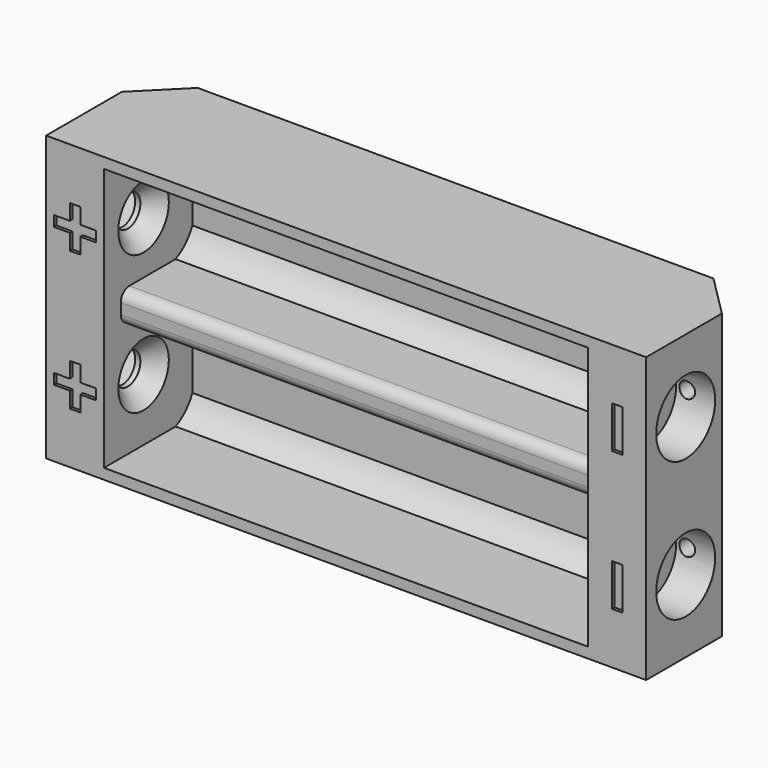
from build123d import *

# Parameters (mm, degrees)
F0_W          = 57
F0_H          = 27
F0_W_2        = 46
F0_H_2        = 25
F1_DEPTH      = 13
F2_DEPTH      = 2.5
F3_W          = 10
F3_H          = 3
F4_DEPTH      = 46
F5_R          = 1.5
F6_DEPTH      = 5.501
F6_DEPTH_BACK = 51.501
F7_SIZE       = 1.5
F8_R          = 1.5
F9_DEPTH      = 3.5
F10_R         = 3.5
F10_R_2       = 1.5
F11_DEPTH     = 3.7
F13_DEPTH     = 46
F14_R         = 1.2
F15_DEPTH     = 57.001
F16_R         = 0.75
F17_DEPTH     = 6
F18_T1_DEPTH  = 47.5734639037
F19_W         = 1
F19_H         = 4
F19_H_2       = 1.5
F19_W_2       = 1.5
F19_H_3       = 1
F20_DEPTH     = 0.3
F21_R         = 1


# Not quite as in the source:
# - a fillet or chamfer that OpenCascade refuses, or shapes differently, is made with other operations: its cross-section is extruded or revolved along the edge and cut away or added


with BuildPart() as f1:
    # F0 (on Front) → F1 (new body)
    with BuildSketch(Plane.XZ):
        Rectangle(F0_W, F0_H)
        Rectangle(F0_W_2, F0_H_2, mode=Mode.SUBTRACT)
    extrude(amount=F1_DEPTH)

    # F0 (on Front) → F2 (join)
    with BuildSketch(Plane.XZ):
        Rectangle(F0_W_2, F0_H_2)
    extrude(amount=F2_DEPTH)

    # F3 (on face) → F4 (join, through all)
    with BuildSketch(Plane.YZ.offset(-23)):
        with Locations((-6, 0)):
            Rectangle(F3_W, F3_H)
    extrude(amount=F4_DEPTH)

    # F5 (on face) → F6 (cut, two sides)
    with BuildSketch(Plane.YZ.offset(-23)) as f6_sk:
        with Locations((-8.3, 6.6)):
            Circle(F5_R)
        with Locations((-8.3, -6.6)):
            Circle(F5_R)
    extrude(amount=-F6_DEPTH, mode=Mode.SUBTRACT)
    extrude(f6_sk.sketch, amount=F6_DEPTH_BACK, mode=Mode.SUBTRACT)

    # F7
    f7_edges = [f1.edges().sort_by_distance(p)[0] for p in [
        (-23, -9.8, 6.6),
        (-23, -9.8, -6.6),
        (23, -9.8, 6.6),
        (23, -9.8, -6.6),
    ]]
    chamfer(f7_edges, length=F7_SIZE)

    # F8 (on face) → F9 (cut)
    with BuildSketch(Plane(origin=(-28.5, 0, 0), x_dir=(0, -1, 0), z_dir=(-1, 0, 0))):
        Polygon((6.5679491924, -3.6), (4.8358983849, -6.6), (6.5679491924, -9.6), (10.0320508076, -9.6), (11.7641016151, -6.6), (10.0320508076, -3.6), align=None)
        with Locations((8.3, -6.6)):
            Circle(F8_R, mode=Mode.SUBTRACT)
        Polygon((10.0320508076, 9.6), (6.5679491924, 9.6), (4.8358983849, 6.6), (6.5679491924, 3.6), (10.0320508076, 3.6), (11.7641016151, 6.6), align=None)
        with Locations((8.3, 6.6)):
            Circle(F8_R, mode=Mode.SUBTRACT)
        with Locations((8.3, 6.6)):
            Circle(F8_R)
    extrude(amount=-F9_DEPTH, mode=Mode.SUBTRACT)

    # F10 (on face) → F11 (cut)
    with BuildSketch(Plane.YZ.offset(28.5)):
        with Locations((-8.3, 6.6)):
            Circle(F10_R)
        with Locations((-8.3, 6.6)):
            Circle(F10_R_2, mode=Mode.SUBTRACT)
        with Locations((-8.3, -6.6)):
            Circle(F10_R)
        with Locations((-8.3, -6.6)):
            Circle(F10_R_2, mode=Mode.SUBTRACT)
    extrude(amount=-F11_DEPTH, mode=Mode.SUBTRACT)

    # F12 (on face) → F13 (join, through all)
    with BuildSketch(Plane.YZ.offset(-23)):
        with BuildLine():
            Line((-2.5, -12.5), (-2.5, -10.5))
            ThreePointArc((-2.5, -10.5), (-3.3173241863, -11.6826758137), (-4.5, -12.5))
            Line((-4.5, -12.5), (-2.5, -12.5))
        make_face()
        with BuildLine():
            ThreePointArc((-4.5, -1.5), (-3.3173241863, -2.3173241863), (-2.5, -3.5))
            Line((-2.5, -3.5), (-2.5, -1.5))
            Line((-2.5, -1.5), (-4.5, -1.5))
        make_face()
        with BuildLine():
            Line((-2.5, 12.5), (-4.5, 12.5))
            ThreePointArc((-4.5, 12.5), (-3.3173241863, 11.6826758137), (-2.5, 10.5))
            Line((-2.5, 10.5), (-2.5, 12.5))
        make_face()
        with BuildLine():
            ThreePointArc((-2.5, 3.5), (-3.3173241863, 2.3173241863), (-4.5, 1.5))
            Line((-4.5, 1.5), (-2.5, 1.5))
            Line((-2.5, 1.5), (-2.5, 3.5))
        make_face()
    extrude(amount=F13_DEPTH)

    # F14 (on face) → F15 (cut, through all)
    with BuildSketch(Plane.YZ.offset(28.5)):
        with Locations((-1.55, 0)):
            Circle(F14_R)
    extrude(amount=-F15_DEPTH, mode=Mode.SUBTRACT)

    # F16 (on face) → F17 (cut)
    with BuildSketch(Plane(origin=(0, 0, 0), x_dir=(-1, 0, 0), z_dir=(0, 1, 0))):
        with Locations((-25.85, -6.6)):
            Circle(F16_R)
        with Locations((-25.85, 6.6)):
            Circle(F16_R)
        with Locations((25.85, 6.6)):
            Circle(F16_R)
        with Locations((25.85, -6.6)):
            Circle(F16_R)
    extrude(amount=-F17_DEPTH, mode=Mode.SUBTRACT)

    # F18: chamfer of 4 on 2 edges, made by hand

    # F18_s2 → F18_t1 (cut)
    with BuildSketch(Plane.XY.offset(-23.7867319519)):
        Polygon((24.5, 0), (28.5, -4), (28.5, 0), align=None)
        Polygon((-28.5, -4), (-24.5, 0), (-28.5, 0), align=None)
    extrude(amount=F18_T1_DEPTH, mode=Mode.SUBTRACT)

    # F19 (on face) → F20 (cut)
    with BuildSketch(Plane.XZ.offset(13)):
        with Locations((25.75, -6.6)):
            Rectangle(F19_W, F19_H)
        with Locations((25.75, 6.6)):
            Rectangle(F19_W, F19_H)
        with Locations((-25.75, 5.35)):
            Rectangle(F19_W, F19_H_2)
        with Locations((-27, 6.6)):
            Rectangle(F19_W_2, F19_H_3)
        with Locations((-25.75, 6.6)):
            Rectangle(F19_W, F19_H_3)
        with Locations((-24.5, 6.6)):
            Rectangle(F19_W_2, F19_H_3)
        with Locations((-25.75, 7.85)):
            Rectangle(F19_W, F19_H_2)
        with Locations((-25.75, -5.35)):
            Rectangle(F19_W, F19_H_2)
        with Locations((-24.5, -6.6)):
            Rectangle(F19_W_2, F19_H_3)
        with Locations((-25.75, -6.6)):
            Rectangle(F19_W, F19_H_3)
        with Locations((-27, -6.6)):
            Rectangle(F19_W_2, F19_H_3)
        with Locations((-25.75, -7.85)):
            Rectangle(F19_W, F19_H_2)
    extrude(amount=-F20_DEPTH, mode=Mode.SUBTRACT)

    # F21
    f21_edges = [f1.edges().sort_by_distance(p)[0] for p in [
        (0, -11, -1.5),
        (0, -11, 1.5),
    ]]
    fillet(f21_edges, radius=F21_R)


solid = f1.part
